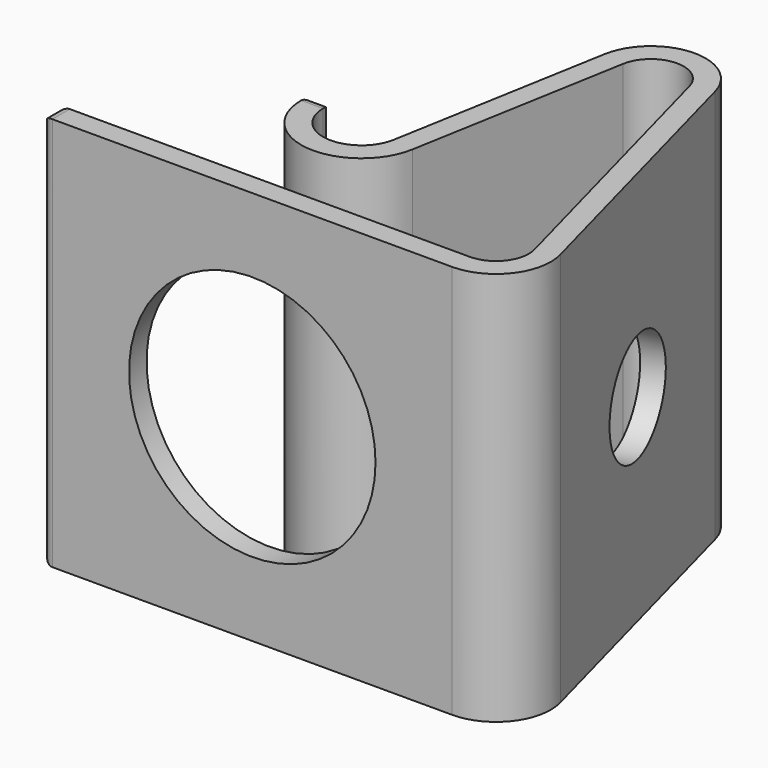
from build123d import *

# Parameters (mm, degrees)
F1_DEPTH = 72
F2_R     = 1.99999
F3_R     = 1.99999
F4_R     = 10
F5_DEPTH = 5
F8_R     = 22.5
F9_DEPTH = 5


# Not quite as in the source:
# - a fillet or chamfer is up to 0.001 mm smaller than in the source, because OpenCascade refuses the exact size
# - a feature of the source that left no trace in its solid (it failed there, or was rolled back) is left out


with BuildPart() as f1:
    # F0 (on Top) → F1 (new body)
    with BuildSketch(Plane.XY):
        with BuildLine():
            Line((-9.8480775301, 1.7364817767), (-16.7940046368, -37.6558283438))
            ThreePointArc((-16.7940046368, -37.6558283438), (-24.2977491071, -43.4136539868), (-30.6876589079, -36.4402911002))
            Line((-30.6876589079, -36.4402911002), (-30.6876589079, -34.4402911002))
            Line((-30.6876589079, -34.4402911002), (-34.6876589079, -34.4402911002))
            Line((-34.6876589079, -34.4402911002), (-34.6876589079, -36.4402911002))
            ThreePointArc((-34.6876589079, -36.4402911002), (-24.6463720781, -47.3984327792), (-12.8547736248, -38.3504210545))
            Line((-12.8547736248, -38.3504210545), (-5.9088465181, 1.041889066))
            ThreePointArc((-5.9088465181, 1.041889066), (-0.2617163242, 5.9942893295), (5.7955549577, 1.5529142706))
            Line((5.7955549577, 1.5529142706), (20.0306024384, -51.5730061753))
            ThreePointArc((20.0306024384, -51.5730061753), (18.9951675224, -56.77848902), (14.2350474806, -59.1259204459))
            Line((14.2350474806, -59.1259204459), (-60.7649525194, -59.1259204459))
            Line((-60.7649525194, -59.1259204459), (-60.7649525194, -63.1259204459))
            Line((-60.7649525194, -63.1259204459), (14.2350474806, -63.1259204459))
            ThreePointArc((14.2350474806, -63.1259204459), (22.1685808836, -59.213534736), (23.8943057435, -50.5377299949))
            Line((23.8943057435, -50.5377299949), (9.6592582629, 2.588190451))
            ThreePointArc((9.6592582629, 2.588190451), (-0.4361938737, 9.9904822158), (-9.8480775301, 1.7364817767))
        make_face()
    extrude(amount=F1_DEPTH)

    # F2 (radius 2 in the source; OpenCascade refuses exactly that, so slightly less here)
    f2_edges = [f1.edges().sort_by_distance(p)[0] for p in [
        (-30.687659, -34.440291, 36),
        (-34.687659, -34.440291, 36),
        (-32.687659, -34.440291, 0),
        (-32.687659, -34.440291, 72),
    ]]
    fillet(f2_edges, radius=F2_R)

    # F3 (radius 2 in the source; OpenCascade refuses exactly that, so slightly less here)
    f3_edges = [f1.edges().sort_by_distance(p)[0] for p in [
        (-60.764953, -59.12592, 36),
        (-60.764953, -63.12592, 36),
        (-60.764953, -61.12592, 0),
        (-60.764953, -61.12592, 72),
    ]]
    fillet(f3_edges, radius=F3_R)

    # F4 (on face) → F5 (cut)
    with BuildSketch(Plane(origin=(9.6592582629, 2.588190451, 0), x_dir=(-0.2588190451, 0.9659258263, 0), z_dir=(0.9659258263, 0.2588190451, 0))):
        with Locations((-27.5, 36)):
            Circle(F4_R)
    extrude(amount=-F5_DEPTH, mode=Mode.SUBTRACT)

    # F8 (on face) → F9 (cut)
    with BuildSketch(Plane.XZ.offset(63.1259204459)):
        with Locations((-22.2649525194, 36)):
            Circle(F8_R)
    extrude(amount=-F9_DEPTH, mode=Mode.SUBTRACT)


solid = f1.part
